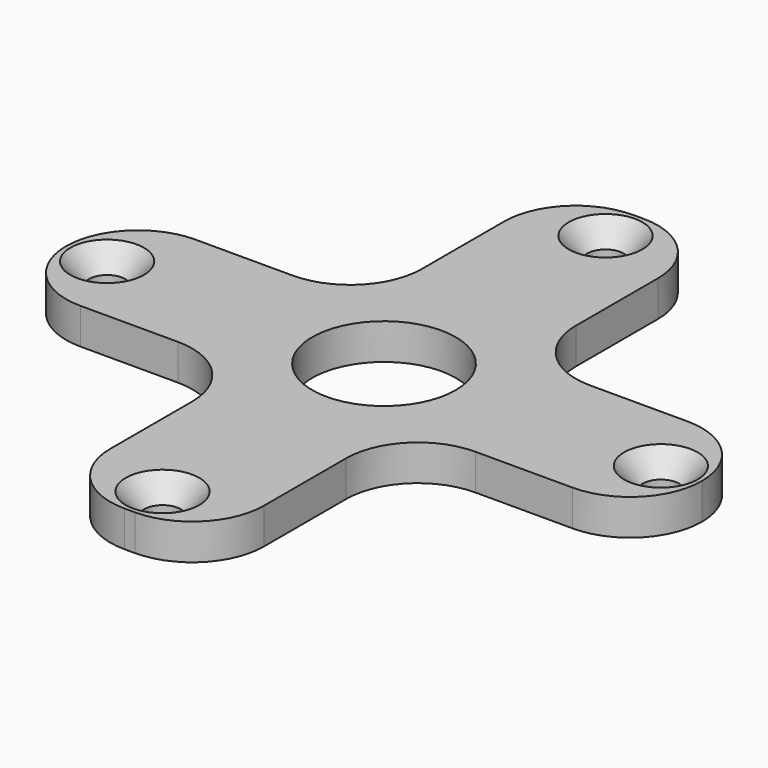
from build123d import *

# Parameters (mm, degrees)
F0_W           = 78.74
F0_H           = 17.78
F1_DEPTH       = 4.445
F2_W           = 19.05
F2_H           = 78.74
F3_DEPTH       = 4.445
F4_R           = 8.88999
F6_D           = 4.4958
F6_CSINK_D     = 9.1186
F6_CSINK_ANGLE = 82
F7_R           = 8.89
F8_DEPTH       = 4.446


# Not quite as in the source:
# - a fillet or chamfer is up to 0.001 mm smaller than in the source, because OpenCascade refuses the exact size


with BuildPart() as f1:
    # F0 (on Top) → F1 (new body)
    with BuildSketch(Plane.XY):
        Rectangle(F0_W, F0_H)
    extrude(amount=F1_DEPTH)

    # F2 (on Top) → F3 (join, through all)
    with BuildSketch(Plane.XY):
        Rectangle(F2_W, F2_H)
    extrude(amount=F3_DEPTH)

    # F4 (radius 8.89 in the source; OpenCascade refuses exactly that, so slightly less here)
    f4_edges = [f1.edges().sort_by_distance(p)[0] for p in [
        (9.525, -39.37, 2.2225),
        (-9.525, -39.37, 2.2225),
        (39.37, -8.89, 2.2225),
        (39.37, 8.89, 2.2225),
        (9.525, 39.37, 2.2225),
        (-39.37, -8.89, 2.2225),
        (-39.37, 8.89, 2.2225),
        (-9.525, 8.89, 2.2225),
        (-9.525, 39.37, 2.2225),
        (-9.525, -8.89, 2.2225),
        (9.525, -8.89, 2.2225),
        (9.525, 8.89, 2.2225),
    ]]
    fillet(f4_edges, radius=F4_R)

    # F6 (through all)
    with Locations(Plane.XY.offset(4.445)):
        with Locations((34.29, 0), (0, -34.29), (-34.29, 0), (0, 34.29)):
            CounterSinkHole(F6_D / 2, F6_CSINK_D / 2, counter_sink_angle=F6_CSINK_ANGLE)

    # F7 (on Top) → F8 (cut, through all)
    with BuildSketch(Plane.XY):
        Circle(F7_R)
    extrude(amount=F8_DEPTH, mode=Mode.SUBTRACT)


solid = f1.part
